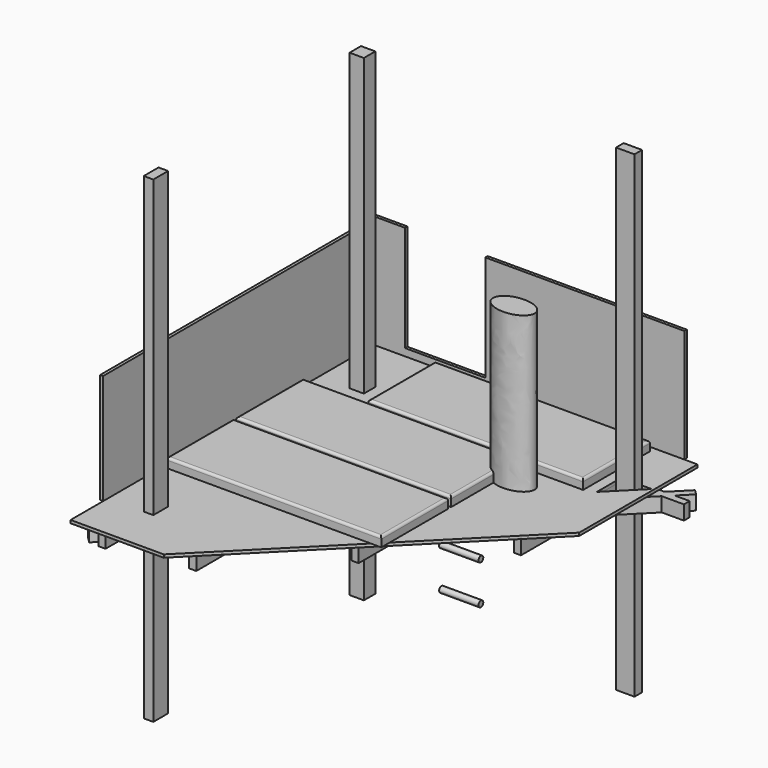
from build123d import *

# Parameters (mm, degrees)
F0_W      = 80
F0_H      = 155
F1_DEPTH  = 4000
F0_W_2    = 120
F0_H_2    = 120
F0_W_3    = 155
F0_H_3    = 80
F3_W      = 600
F3_H      = 60
F3_W_2    = 60
F3_H_2    = 440
F3_W_3    = 240
F3_W_4    = 700
F4_DEPTH  = 120
F5_W      = 200
F5_H      = 400
F5_W_2    = 270.1964569092
F5_W_3    = 700
F5_W_4    = 600
F6_DEPTH  = 25
F7_W      = 1800
F7_H      = 700
F8_DEPTH  = 80
F9_R      = 20
F9_2_R    = 20
F9_3_R    = 20
F13_DEPTH = 1300
F15_DEPTH = 25
F17_DEPTH = 25
F21_W     = 673.2819676399
F21_H     = 887.2460126877
F22_DEPTH = 25
F23_R     = 25
F24_DEPTH = 330


# Not quite as in the source:
# - a feature names something its author has since deleted; it is built from what else it names


with BuildPart() as f1:
    # F0 (on Top) → F1 (new body)
    with BuildSketch(Plane.XY):
        with Locations((80, -2247.5)):
            Rectangle(F0_W, F0_H)
    extrude(amount=F1_DEPTH)


with BuildPart() as f1b:
    # F0 (on Top) → F1, piece 2 (new body)
    with BuildSketch(Plane.XY):
        with Locations((60, -60)):
            Rectangle(F0_W_2, F0_H_2)
    extrude(amount=F1_DEPTH)


with BuildPart() as f1c:
    # F0 (on Top) → F1, piece 3 (new body)
    with BuildSketch(Plane.XY):
        with Locations((2277.5, -40)):
            Rectangle(F0_W_3, F0_H_3)
    extrude(amount=F1_DEPTH)


with BuildPart() as f4:
    # F3 (on offset) → F4 (new body)
    with BuildSketch(Plane.XY.offset(1500)):
        Polygon((-60, -2590.8482220543), (0, -2530.5797656785), (0, -2445.5369127517), (-60, -2505.8053691275), align=None)
        Polygon((-60, -2675), (0, -2675), (0, -2530.5797656785), (-60, -2590.8482220543), align=None)
        Polygon((-140, -2671.2061638888), (-60, -2590.8482220543), (-60, -2505.8053691275), (-182.5210027427, -2628.8745642763), align=None)
        Polygon((0, -2445.5369127517), (0, -2530.5797656785), (600, -1927.8952019201), (600, -1842.8523489933), align=None)
        Polygon((-60, -2505.8053691275), (0, -2445.5369127517), (0, 0), (-60, 0), align=None)
        with Locations((300, 30)):
            Rectangle(F3_W, F3_H)
        Polygon((2579.0404348737, 60), (2519.3076954527, 0), (2705, 0), (2705, 60), align=None)
        Polygon((2494.3763919822, 60), (2579.0404348737, 60), (2678.5950005752, 160), (2636.0739978325, 202.3315996125), align=None)
        Polygon((2434.6436525612, 0), (2519.3076954527, 0), (2579.0404348737, 60), (2494.3763919822, 60), align=None)
        with Locations((-30, 280)):
            Rectangle(F3_W_2, F3_H_2)
        with Locations((-180, 30)):
            Rectangle(F3_W_3, F3_H)
        with Locations((-30, 30)):
            Rectangle(F3_W_2, F3_H)
        Polygon((600, 0), (600, -1842.8523489933), (660, -1782.5838926174), (660, 0), align=None)
        Polygon((660, -1867.6267455442), (600, -1927.8952019201), (600, -2550), (660, -2550), align=None)
        Polygon((1420, -1104.2262981169), (1360, -1164.4947544928), (1360, -1800), (1420, -1800), align=None)
        Polygon((1360, 0), (1360, -1079.451901566), (1420, -1019.1834451902), (1420, 0), align=None)
        Polygon((660, -1782.5838926174), (660, -1867.6267455442), (1360, -1164.4947544928), (1360, -1079.451901566), align=None)
        Polygon((1420, -1019.1834451902), (1420, -1104.2262981169), (2120, -401.0943070655), (2120, -316.0514541387), align=None)
        Polygon((2180, -340.8258506896), (2120, -401.0943070655), (2120, -1050), (2180, -1050), align=None)
        Polygon((600, -1842.8523489933), (600, -1927.8952019201), (660, -1867.6267455442), (660, -1782.5838926174), align=None)
        Polygon((1360, -1079.451901566), (1360, -1164.4947544928), (1420, -1104.2262981169), (1420, -1019.1834451902), align=None)
        Polygon((2120, -316.0514541387), (2120, -401.0943070655), (2180, -340.8258506896), (2180, -255.7829977629), align=None)
        Polygon((2180, -255.7829977629), (2180, -340.8258506896), (2519.3076954527, 0), (2434.6436525612, 0), align=None)
        Polygon((2180, 60), (2180, 0), (2434.6436525612, 0), (2494.3763919822, 60), align=None)
        with Locations((2150, 30)):
            Rectangle(F3_W_2, F3_H)
        Polygon((2120, 0), (2120, -316.0514541387), (2180, -255.7829977629), (2180, 0), align=None)
        with Locations((2150, 280)):
            Rectangle(F3_W_2, F3_H_2)
        with Locations((1390, 280)):
            Rectangle(F3_W_2, F3_H_2)
        with Locations((1390, 30)):
            Rectangle(F3_W_2, F3_H)
        with Locations((1010, 30)):
            Rectangle(F3_W_4, F3_H)
        with Locations((630, 30)):
            Rectangle(F3_W_2, F3_H)
        with Locations((630, 280)):
            Rectangle(F3_W_2, F3_H_2)
        with Locations((1770, 30)):
            Rectangle(F3_W_4, F3_H)
    extrude(amount=-F4_DEPTH)


with BuildPart() as f6:
    # F5 (on face) → F6 (new body)
    with BuildSketch(Plane.XY.offset(1500)):
        with Locations((-160, 260)):
            Rectangle(F5_W, F5_H)
        Polygon((-60, 60), (-260, 60), (-260, 0), (-60, 0), (-60, -2505.8053691275), (-182.5210027427, -2628.8745642763), (-140, -2671.2061638888), (-60, -2590.8482220543), (-60, -2675), (0, -2675), (0, -2530.5797656785), (600, -1927.8952019201), (600, -2550), (660, -2550), (660, -1867.6267455442), (1360, -1164.4947544928), (1360, -1800), (1420, -1800), (1420, -1104.2262981169), (2120, -401.0943070655), (2120, -1050), (2179.5184463486, -1050), (2180, -1049.5162917462), (2180, -340.8258506896), (2450.1964569092, -69.4204610874), (2450.1964569092, 60), (2180, 60), (2180, 460), (2120, 460), (2120, 60), (1420, 60), (1420, 460), (1360, 460), (1360, 60), (660, 60), (660, 460), (600, 460), (600, 60), (0, 60), (0, 460), (-60, 460), align=None)
        Polygon((0, -2445.5369127517), (0, 0), (600, 0), (600, -1842.8523489933), align=None, mode=Mode.SUBTRACT)
        Polygon((1360, -1079.451901566), (660, -1782.5838926174), (660, 0), (1360, 0), align=None, mode=Mode.SUBTRACT)
        Polygon((1420, 0), (2120, 0), (2120, -316.0514541387), (1420, -1019.1834451902), align=None, mode=Mode.SUBTRACT)
        Polygon((2180, 0), (2434.6436525612, 0), (2180, -255.7829977629), align=None, mode=Mode.SUBTRACT)
        with Locations((2315.0982284546, 260)):
            Rectangle(F5_W_2, F5_H)
        Polygon((-60, 0), (-260, 0), (-260, -2716.2301540375), (520.7102529082, -2716.2301540375), (2179.5184463486, -1050), (2120, -1050), (2120, -401.0943070655), (1420, -1104.2262981169), (1420, -1800), (1360, -1800), (1360, -1164.4947544928), (660, -1867.6267455442), (660, -2550), (600, -2550), (600, -1927.8952019201), (0, -2530.5797656785), (0, -2675), (-60, -2675), (-60, -2590.8482220543), (-140, -2671.2061638888), (-182.5210027427, -2628.8745642763), (-60, -2505.8053691275), align=None)
        Polygon((2180, -340.8258506896), (2180, -1049.5162917462), (2450.1964569092, -778.1109021439), (2450.1964569092, -69.4204610874), align=None)
        Polygon((660, 0), (660, -1782.5838926174), (1360, -1079.451901566), (1360, 0), align=None)
        Polygon((2120, -316.0514541387), (2120, 0), (1420, 0), (1420, -1019.1834451902), align=None)
        with Locations((1770, 260)):
            Rectangle(F5_W_3, F5_H)
        with Locations((1010, 260)):
            Rectangle(F5_W_3, F5_H)
        with Locations((300, 260)):
            Rectangle(F5_W_4, F5_H)
        Polygon((600, 0), (0, 0), (0, -2445.5369127517), (600, -1842.8523489933), align=None)
    extrude(amount=F6_DEPTH)


with BuildPart() as f8:
    # F7 (on face) → F8 (new body)
    with BuildSketch(Plane.XY.offset(1525)):
        with Locations((1192.6203727722, 60)):
            Rectangle(F7_W, F7_H)
    extrude(amount=F8_DEPTH)

    # F9#3
    f9_3_edges = [f8.edges().sort_by_distance(p)[0] for p in [
        (1192.620373, -290, 1605),
        (292.620373, 60, 1605),
        (1192.620373, 410, 1605),
        (2092.620373, 60, 1605),
    ]]
    fillet(f9_3_edges, radius=F9_3_R)


with BuildPart() as f8b:
    # F7 (on face) → F8, piece 2 (new body)
    with BuildSketch(Plane.XY.offset(1525)):
        with Locations((670, -670)):
            Rectangle(F7_W, F7_H)
    extrude(amount=F8_DEPTH)

    # F9#2
    f9_2_edges = [f8b.edges().sort_by_distance(p)[0] for p in [
        (670, -1020, 1605),
        (1570, -670, 1605),
        (670, -320, 1605),
        (-230, -670, 1605),
    ]]
    fillet(f9_2_edges, radius=F9_2_R)


with BuildPart() as f8c:
    # F7 (on face) → F8, piece 3 (new body)
    with BuildSketch(Plane.XY.offset(1525)):
        Polygon((1570, -1050), (-230, -1050), (-230, -1750), (1482.6364864377, -1750), (1570, -1662.2455982339), align=None)
        Polygon((1570, -1750), (1570, -1662.2455982339), (1482.6364864377, -1750), align=None)
    extrude(amount=F8_DEPTH)

    # F9
    f9_edges = [f8c.edges().sort_by_distance(p)[0] for p in [
        (670, -1750, 1605),
        (-230, -1400, 1605),
        (670, -1050, 1605),
        (1570, -1400, 1605),
    ]]
    fillet(f9_edges, radius=F9_R)


with BuildPart() as f13:
    # F12 (on face) → F13 (new body)
    with BuildSketch(Plane.XY.offset(1525)):
        with BuildLine():
            add(Edge.make_bspline(
                [(1842.9663658142, -484.9302768707), (1842.9663658142, -294.4046880382), (1580.4663658142, -389.6674824544), (1317.9663658142, -484.9302768707), (1580.4663658142, -580.193071287), (1842.9663658142, -675.4558657033), (1842.9663658142, -484.9302768707)],
                knots=[0, 0, 0, 2.0943951024, 2.0943951024, 4.1887902048, 4.1887902048, 6.2831853072, 6.2831853072, 6.2831853072], degree=2, weights=[1, 0.5, 1, 0.5, 1, 0.5, 1]))
        make_face()
    extrude(amount=F13_DEPTH)


with BuildPart() as f15:
    # F14 (on face) → F15 (new body)
    with BuildSketch(Plane(origin=(0, 460, 0), x_dir=(-1, 0, 0), z_dir=(0, 1, 0))):
        Polygon((-2341.2070274353, 1500), (-2341.2070274353, 1426.1865615845), (339.0676081181, 1426.1865615845), (339.0676081181, 2473.1640815735), (-2341.2070274353, 2473.1640815735), (-2341.2070274353, 1525), (260, 1525), (260, 1500), align=None)
    extrude(amount=F15_DEPTH)

    # F21 (on face) → F22 (cut)
    with BuildSketch(Plane(origin=(0, 485, 0), x_dir=(-1, 0, 0), z_dir=(0, 1, 0))):
        with Locations((-336.64098382, 2029.5410752296)):
            Rectangle(F21_W, F21_H)
    extrude(amount=-F22_DEPTH, mode=Mode.SUBTRACT)


with BuildPart() as f17:
    # F16 (on face) → F17 (new body)
    with BuildSketch(Plane(origin=(-260, 0, 0), x_dir=(0, -1, 0), z_dir=(-1, 0, 0))):
        Polygon((-460.2313935757, 2447.8528499603), (-460.2313935757, 1443.4218406677), (2374.6094703674, 1443.4218406677), (2374.6094703674, 1500), (-460, 1500), (-460, 1525), (2374.6094703674, 1525), (2374.6094703674, 2447.8528499603), align=None)
    extrude(amount=F17_DEPTH)


with BuildPart() as f24:
    # F23 (on face) → F24 (new body)
    with BuildSketch(Plane(origin=(600, 0, 0), x_dir=(0, -1, 0), z_dir=(-1, 0, 0))):
        with Locations((-505.343735218, 1196.3505744934)):
            Circle(F23_R)
    extrude(amount=F24_DEPTH)


with BuildPart() as f24b:
    # F23 (on face) → F24, piece 2 (new body)
    with BuildSketch(Plane(origin=(600, 0, 0), x_dir=(0, -1, 0), z_dir=(-1, 0, 0))):
        with Locations((-505.343735218, 866.3505744934)):
            Circle(F23_R)
    extrude(amount=F24_DEPTH)


with BuildPart() as f24c:
    # F23 (on face) → F24, piece 3 (new body)
    with BuildSketch(Plane(origin=(600, 0, 0), x_dir=(0, -1, 0), z_dir=(-1, 0, 0))):
        with Locations((-505.343735218, 536.3505744934)):
            Circle(F23_R)
    extrude(amount=F24_DEPTH)


with BuildPart() as f24d:
    # F23 (on face) → F24, piece 4 (new body)
    with BuildSketch(Plane(origin=(600, 0, 0), x_dir=(0, -1, 0), z_dir=(-1, 0, 0))):
        with Locations((-505.343735218, 206.3505744934)):
            Circle(F23_R)
    extrude(amount=F24_DEPTH)


with BuildPart() as f24e:
    # F23 (on face) → F24, piece 5 (new body)
    with BuildSketch(Plane(origin=(600, 0, 0), x_dir=(0, -1, 0), z_dir=(-1, 0, 0))):
        with Locations((-505.343735218, -123.6494255066)):
            Circle(F23_R)
    extrude(amount=F24_DEPTH)


solid = Compound([f1.part, f1b.part, f1c.part, f4.part, f6.part, f8.part, f8b.part, f8c.part, f13.part, f15.part, f17.part, f24.part, f24b.part, f24c.part, f24d.part, f24e.part])
